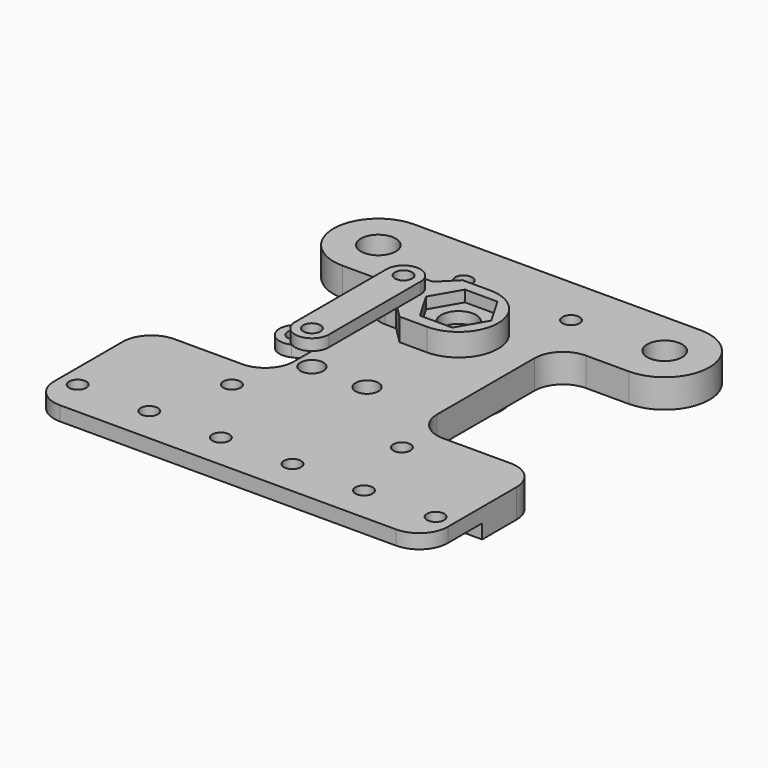
from build123d import *

# Parameters (mm, degrees)
F0_W      = 69.85
F0_H      = 73.025
F1_DEPTH  = 5.08
F2_W      = 12.7
F2_H      = 2.54
F3_DEPTH  = 69.851
F4_R      = 3.1
F4_R_2    = 6
F5_DEPTH  = 5.08
F6_R      = 5.08
F8_R      = 17.4625
F9_DEPTH  = 4
F10_R     = 3.1
F11_DEPTH = 25.4
F12_R     = 3.1
F14_DEPTH = 1.5
F15_R     = 1.524
F16_DEPTH = 4
F18_DEPTH = 4
F19_R     = 1.524
F20_DEPTH = 2
F13_R     = 1.524
F21_DEPTH = 2.54
F22_R     = 1.524
F22_R_2   = 3.1
F23_DEPTH = 4
F25_DEPTH = 2
F27_DEPTH = 4
F28_R     = 2.032
F29_DEPTH = 5.08
F30_R     = 1.524
F31_DEPTH = 5.08
F32_R     = 2.794
F33_DEPTH = 2.54
F34_R     = 2.794
F35_DEPTH = 2.54
F36_R     = 1.524
F37_DEPTH = 2


# Not quite as in the source:
# - a feature names something its author has since deleted; it is built from what else it names


with BuildPart() as f1:
    # F0 (on Top) → F1 (new body)
    with BuildSketch(Plane.XY):
        Rectangle(F0_W, F0_H)
    extrude(amount=F1_DEPTH)

    # F2 (on face) → F3 (cut, through all)
    with BuildSketch(Plane(origin=(-34.925, 0, 0), x_dir=(0, -1, 0), z_dir=(-1, 0, 0))):
        with Locations((30.1625, 1.27)):
            Rectangle(F2_W, F2_H)
    extrude(amount=-F3_DEPTH, mode=Mode.SUBTRACT)

    # F4 (on face) → F5 (cut, through all)
    with BuildSketch(Plane(origin=(0, 0, 0), x_dir=(1, 0, 0), z_dir=(0, 0, -1))):
        with Locations((-25.4, -28.575)):
            Circle(F4_R)
        with Locations((0, -14.6304)):
            Circle(F4_R_2)
        with Locations((25.4, -28.575)):
            Circle(F4_R)
        with BuildLine():
            Line((-34.925, -36.5125), (-25.4, -36.5125))
            ThreePointArc((-25.4, -36.5125), (-33.3375, -28.575), (-25.4, -20.6375))
            Line((-25.4, -20.6375), (-12.7, -20.6375))
            Line((-12.7, -20.6375), (-12.7, 11.1125))
            Line((-12.7, 11.1125), (-34.925, 11.1125))
            Line((-34.925, 11.1125), (-34.925, -36.5125))
        make_face()
        with BuildLine():
            ThreePointArc((25.4, -20.6375), (33.3375, -28.575), (25.4, -36.5125))
            Line((25.4, -36.5125), (34.925, -36.5125))
            Line((34.925, -36.5125), (34.925, 11.1125))
            Line((34.925, 11.1125), (12.7, 11.1125))
            Line((12.7, 11.1125), (12.7, -20.6375))
            Line((12.7, -20.6375), (25.4, -20.6375))
        make_face()
    extrude(amount=-F5_DEPTH, mode=Mode.SUBTRACT)

    # F6
    f6_edges = [f1.edges().sort_by_distance(p)[0] for p in [
        (-12.7, 20.6375, 2.54),
        (12.7, 20.6375, 2.54),
        (12.7, -11.1125, 2.54),
        (-12.7, -11.1125, 2.54),
        (34.925, -11.1125, 2.54),
        (-34.925, -11.1125, 2.54),
        (-34.925, -36.5125, 3.81),
        (34.925, -36.5125, 3.81),
    ]]
    fillet(f6_edges, radius=F6_R)

    # F13 (on face) → F21 (cut, through all)
    with BuildSketch(Plane(origin=(0, 0, 2.54), x_dir=(1, 0, 0), z_dir=(0, 0, -1))):
        with Locations((-31.75, 30.1625)):
            Circle(F13_R)
        with Locations((-19.05, 30.1625)):
            Circle(F13_R)
        with Locations((-6.35, 30.1625)):
            Circle(F13_R)
        with Locations((6.35, 30.1625)):
            Circle(F13_R)
        with Locations((19.05, 30.1625)):
            Circle(F13_R)
        with Locations((31.75, 30.1625)):
            Circle(F13_R)
    extrude(amount=-F21_DEPTH, mode=Mode.SUBTRACT)

    # F28 (on face) → F29 (cut, through all)
    with BuildSketch(Plane.XY.offset(5.08)):
        with Locations((0, -5.6896)):
            Circle(F28_R)
        with Locations((-9.779, -5.6896)):
            Circle(F28_R)
    extrude(amount=-F29_DEPTH, mode=Mode.SUBTRACT)

    # F30 (on face) → F31 (cut, through all)
    with BuildSketch(Plane.XY.offset(5.08)):
        with Locations((15.08125, -16.8021)):
            Circle(F30_R)
        with Locations((-15.08125, -16.8021)):
            Circle(F30_R)
        with Locations((-9.525, 27.6479)):
            Circle(F30_R)
        with Locations((9.525, 27.6479)):
            Circle(F30_R)
    extrude(amount=-F31_DEPTH, mode=Mode.SUBTRACT)


with BuildPart() as f9:
    # F8 (on offset) → F9 (new body)
    with BuildSketch(Plane(origin=(0, 0, -0.381), x_dir=(1, 0, 0), z_dir=(0, 0, -1))):
        with Locations((0, -14.6304)):
            Circle(F8_R)
    extrude(amount=F9_DEPTH)

    # F10 (on face) → F11 (cut)
    with BuildSketch(Plane(origin=(0, 0, -4.381), x_dir=(1, 0, 0), z_dir=(0, 0, -1))):
        with Locations((0, -14.6304)):
            Circle(F10_R)
    extrude(amount=-F11_DEPTH, mode=Mode.SUBTRACT)

    # F12 (on face) → F14 (cut)
    with BuildSketch(Plane(origin=(0, 0, -4.381), x_dir=(1, 0, 0), z_dir=(0, 0, -1))):
        Polygon((5.7735026919, -14.6304), (2.8867513459, -9.6304), (-2.8867513459, -9.6304), (-5.7735026919, -14.6304), (-2.8867513459, -19.6304), (2.8867513459, -19.6304), align=None)
        with Locations((0, -14.6304)):
            Circle(F12_R, mode=Mode.SUBTRACT)
    extrude(amount=-F14_DEPTH, mode=Mode.SUBTRACT)

    # F15 (on face) → F16 (cut, through all)
    with BuildSketch(Plane(origin=(0, 0, -4.381), x_dir=(1, 0, 0), z_dir=(0, 0, -1))):
        with Locations((-3.2870018728, -26.8976579939)):
            Circle(F15_R)
        with Locations((3.2870018728, -26.8976579939)):
            Circle(F15_R)
    extrude(amount=-F16_DEPTH, mode=Mode.SUBTRACT)

    # F17 (on face) → F18 (cut, through all)
    with BuildSketch(Plane(origin=(0, 0, -4.381), x_dir=(1, 0, 0), z_dir=(0, 0, -1))):
        with BuildLine():
            Line((-6.477, -30.8472855595), (-6.477, -18.6444840798))
            ThreePointArc((-6.477, -18.6444840798), (0, -7.0104), (6.477, -18.6444840798))
            Line((6.477, -18.6444840798), (6.477, -30.8472855595))
            ThreePointArc((6.477, -30.8472855595), (14.4575848389, -24.4241299776), (17.4625, -14.6304))
            ThreePointArc((17.4625, -14.6304), (-9.7937299776, -0.1728151611), (-6.477, -30.8472855595))
        make_face()
    extrude(amount=-F18_DEPTH, mode=Mode.SUBTRACT)

    # F34 (on face) → F35 (cut)
    with BuildSketch(Plane.XY.offset(-0.381)):
        with Locations((-3.2870018728, 26.8976579939)):
            Circle(F34_R)
        with Locations((3.2870018728, 26.8976579939)):
            Circle(F34_R)
    extrude(amount=-F35_DEPTH, mode=Mode.SUBTRACT)


with BuildPart() as f20:
    # F19 (on face) → F20 (new body)
    with BuildSketch(Plane(origin=(0, 0, -4.381), x_dir=(1, 0, 0), z_dir=(0, 0, -1))):
        with BuildLine():
            ThreePointArc((-27.4772939699, -11.9271346595), (-31.4814653405, -13.3294939699), (-30.0791060301, -17.3336653405))
            Line((-30.0791060301, -17.3336653405), (-4.5879079029, -29.6009233343))
            ThreePointArc((-4.5879079029, -29.6009233343), (-0.5837365323, -28.1985640239), (-1.9860958427, -24.1943926534))
            Line((-1.9860958427, -24.1943926534), (-27.4772939699, -11.9271346595))
        make_face()
        with Locations((-3.2870018728, -26.8976579939)):
            Circle(F19_R, mode=Mode.SUBTRACT)
        with Locations((-28.7782, -14.6304)):
            Circle(F19_R, mode=Mode.SUBTRACT)
    extrude(amount=F20_DEPTH)


with BuildPart() as f23:
    # F22 (on face) → F23 (new body)
    with BuildSketch(Plane.XY.offset(5.08)):
        with BuildLine():
            Line((0, 21.6304), (-9.779, 21.6304))
            ThreePointArc((-9.779, 21.6304), (-16.779, 14.6304), (-9.779, 7.6304))
            Line((-9.779, 7.6304), (0, 7.6304))
            ThreePointArc((0, 7.6304), (7, 14.6304), (0, 21.6304))
        make_face()
        with Locations((-9.779, 14.6304)):
            Circle(F22_R, mode=Mode.SUBTRACT)
        with Locations((0, 14.6304)):
            Circle(F22_R_2, mode=Mode.SUBTRACT)
    extrude(amount=F23_DEPTH)

    # F24 (on face) → F25 (cut)
    with BuildSketch(Plane.XY.offset(9.08)):
        Polygon((2.8867513459, 19.6304), (-2.8867513459, 19.6304), (-5.7735026919, 14.6304), (-2.8867513459, 9.6304), (2.8867513459, 9.6304), (5.7735026919, 14.6304), align=None)
    extrude(amount=-F25_DEPTH, mode=Mode.SUBTRACT)

    # F26 (on face) → F27 (cut, through all)
    with BuildSketch(Plane.XY.offset(9.08)):
        with BuildLine():
            Line((-7.8255, 10.5664), (-9.779, 10.5664))
            ThreePointArc((-9.779, 10.5664), (-13.843, 14.6304), (-9.779, 18.6944))
            Line((-9.779, 18.6944), (-7.8255, 18.6944))
            Line((-7.8255, 18.6944), (-4.8895, 21.6304))
            Line((-4.8895, 21.6304), (-9.779, 21.6304))
            ThreePointArc((-9.779, 21.6304), (-16.779, 14.6304), (-9.779, 7.6304))
            Line((-9.779, 7.6304), (-4.8895, 7.6304))
            Line((-4.8895, 7.6304), (-7.8255, 10.5664))
        make_face()
    extrude(amount=-F27_DEPTH, mode=Mode.SUBTRACT)

    # F32 (on face) → F33 (cut)
    with BuildSketch(Plane(origin=(0, 0, 5.08), x_dir=(1, 0, 0), z_dir=(0, 0, -1))):
        with Locations((-9.779, -14.6304)):
            Circle(F32_R)
    extrude(amount=-F33_DEPTH, mode=Mode.SUBTRACT)


with BuildPart() as f37:
    # F36 (on face) → F37 (new body)
    with BuildSketch(Plane.XY.offset(9.08)):
        with BuildLine():
            Line((-6.779, -5.6896), (-6.779, 14.6304))
            ThreePointArc((-6.779, 14.6304), (-9.779, 17.6304), (-12.779, 14.6304))
            Line((-12.779, 14.6304), (-12.779, -5.6896))
            ThreePointArc((-12.779, -5.6896), (-9.779, -8.6896), (-6.779, -5.6896))
        make_face()
        with Locations((-9.779, -5.6896)):
            Circle(F36_R, mode=Mode.SUBTRACT)
        with Locations((-9.779, 14.6304)):
            Circle(F36_R, mode=Mode.SUBTRACT)
    extrude(amount=F37_DEPTH)


solid = Compound([f1.part, f9.part, f20.part, f23.part, f37.part])
